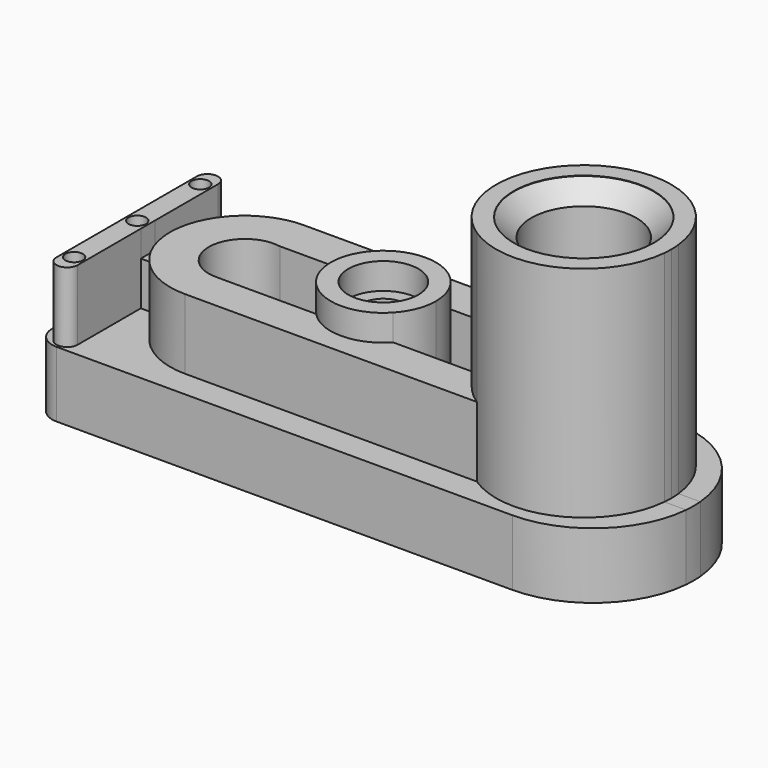
from build123d import *

# Parameters (mm, degrees)
F1_DEPTH  = 15
F0_R      = 2
F2_DEPTH  = 31
F3_DEPTH  = 25
F4_DEPTH  = 31
F0_R_2    = 8
F5_DEPTH  = 37
F0_R_3    = 5
F6_DEPTH  = 31
F0_R_4    = 16
F0_R_5    = 12
F7_DEPTH  = 65
F8_DEPTH  = 65
F10_DEPTH = 15
F11_DEPTH = 15


# Not quite as in the source:
# - a fillet or chamfer that OpenCascade refuses, or shapes differently, is made with other operations: its cross-section is extruded or revolved along the edge and cut away or added
# - a feature names something its author has since deleted; it is built from what else it names


with BuildPart() as f1:
    # F0 (on Top) → F1 (new body)
    with BuildSketch(Plane.XY):
        with BuildLine():
            ThreePointArc((77.4165694517, 2), (70.0412743977, 16.9583212199), (54.4963863199, 23.0000763868))
            Line((54.4963863199, 23.0000763868), (-49.5028280384, 23.0000763868))
            ThreePointArc((-49.5028280384, 23.0000763868), (-53.0386396779, 21.5353325374), (-54.5028279767, 17.9992908068))
            Line((-54.5028279767, 17.9992908068), (-54.4971717765, -18.0008619668))
            ThreePointArc((-54.4971717765, -18.0008619668), (-53.0324279887, -21.5358880263), (-49.4971718382, -23.0000763868))
            Line((-49.4971718382, -23.0000763868), (54.5036136801, -23.0000763868))
            ThreePointArc((54.5036136801, -23.0000763868), (70.024037462, -16.9740969207), (77.4118141054, -2.0537504379))
            Line((77.4118141054, -2.0537504379), (72.4417991653, -2.0537504379))
            ThreePointArc((72.4417991653, -2.0537504379), (61.1210212719, -18.2127692775), (41.4420685321, -16.7940652806))
            Line((41.4420685321, -16.7940652806), (-25.1657858694, -16.7940652806))
            ThreePointArc((-25.1657858694, -16.7940652806), (-36.3795967687, -12.5710150384), (-42.0220562758, -2))
            Line((-42.0220562758, -2), (-47.0725483227, -2))
            Line((-47.0725483227, -2), (-47.0801730056, -20.0009441468))
            ThreePointArc((-47.0801730056, -20.0009441468), (-49.4958146373, -22.4147707226), (-51.9095643269, -19.999052265))
            Line((-51.9095643269, -19.999052265), (-51.8926214772, 20.0009441468))
            ThreePointArc((-51.8926214772, 20.0009441468), (-49.4769799058, 22.4146170129), (-47.0632301559, 19.999052265))
            Line((-47.0632301559, 19.999052265), (-47.0708540375, 2))
            Line((-47.0708540375, 2), (-42.0708540375, 2))
            ThreePointArc((-42.0708540375, 2), (-36.5346224464, 12.8451417707), (-25.1657858694, 17.2059347194))
            Line((-25.1657858694, 17.2059347194), (42.5953938554, 17.2059347194))
            ThreePointArc((42.5953938554, 17.2059347194), (61.6177075826, 17.6666940031), (72.4165694517, 2))
            Line((72.4165694517, 2), (77.4165694517, 2))
        make_face()
    extrude(amount=F1_DEPTH)

    # F0 (on Top) → F2 (join)
    with BuildSketch(Plane.XY):
        with BuildLine():
            Line((-47.0725483227, -2), (-47.0708540375, 2))
            Line((-47.0708540375, 2), (-47.0632301559, 19.999052265))
            ThreePointArc((-47.0632301559, 19.999052265), (-49.4769799058, 22.4146170129), (-51.8926214772, 20.0009441468))
            Line((-51.8926214772, 20.0009441468), (-51.9095643269, -19.999052265))
            ThreePointArc((-51.9095643269, -19.999052265), (-49.4958146373, -22.4147707226), (-47.0801730056, -20.0009441468))
            Line((-47.0801730056, -20.0009441468), (-47.0725483227, -2))
        make_face()
        with Locations((-49.4971718382, -18.0000763868)):
            Circle(F0_R, mode=Mode.SUBTRACT)
        with Locations((-49.4863972414, 0)):
            Circle(F0_R, mode=Mode.SUBTRACT)
        with Locations((-49.5028280384, 18.0000763868)):
            Circle(F0_R, mode=Mode.SUBTRACT)
    extrude(amount=F2_DEPTH)

    # F0 (on Top) → F3 (join)
    with BuildSketch(Plane.XY):
        with BuildLine():
            ThreePointArc((-42.0220562758, -2), (-42.1645209866, -0.0014403371), (-42.0708540375, 2))
            Line((-42.0708540375, 2), (-47.0708540375, 2))
            Line((-47.0708540375, 2), (-47.0725483227, -2))
            Line((-47.0725483227, -2), (-42.0220562758, -2))
        make_face()
    extrude(amount=F3_DEPTH)

    # F0 (on Top) → F4 (join)
    with BuildSketch(Plane.XY):
        with BuildLine():
            ThreePointArc((34.3503431001, 8.1804120839), (37.766383698, 13.3385657076), (42.5953938554, 17.2059347194))
            Line((42.5953938554, 17.2059347194), (-25.1657858694, 17.2059347194))
            ThreePointArc((-25.1657858694, 17.2059347194), (-36.5346224464, 12.8451417707), (-42.0708540375, 2))
            ThreePointArc((-42.0708540375, 2), (-42.1645209866, -0.0014403371), (-42.0220562758, -2))
            ThreePointArc((-42.0220562758, -2), (-36.3795967687, -12.5710150384), (-25.1657858694, -16.7940652806))
            Line((-25.1657858694, -16.7940652806), (41.4420685321, -16.7940652806))
            ThreePointArc((41.4420685321, -16.7940652806), (37.2108856838, -13.0055426049), (34.2152341998, -8.1804120839))
            Line((34.2152341998, -8.1804120839), (15.4548283117, -8.1804120839))
            ThreePointArc((15.4548283117, -8.1804120839), (6.6752578132, -12), (-2.1043126853, -8.1804120839))
            Line((-2.1043126853, -8.1804120839), (-24.9639281544, -8.1804120839))
            ThreePointArc((-24.9639281544, -8.1804120839), (-33.1770221677, 0.8003828075), (-23.5, 8.1804120839))
            Line((-23.5, 8.1804120839), (-2.1043126853, 8.1804120839))
            ThreePointArc((-2.1043126853, 8.1804120839), (6.6752578132, 12), (15.4548283117, 8.1804120839))
            Line((15.4548283117, 8.1804120839), (34.3503431001, 8.1804120839))
        make_face()
    extrude(amount=F4_DEPTH)

    # F0 (on Top) → F5 (join)
    with BuildSketch(Plane.XY):
        with BuildLine():
            ThreePointArc((18.6752578132, 0), (17.8411622992, 4.3957453303), (15.4548283117, 8.1804120839))
            ThreePointArc((15.4548283117, 8.1804120839), (6.6752578132, 12), (-2.1043126853, 8.1804120839))
            ThreePointArc((-2.1043126853, 8.1804120839), (-5.3247421868, 0), (-2.1043126853, -8.1804120839))
            ThreePointArc((-2.1043126853, -8.1804120839), (6.6752578132, -12), (15.4548283117, -8.1804120839))
            ThreePointArc((15.4548283117, -8.1804120839), (17.8411622992, -4.3957453303), (18.6752578132, 0))
        make_face()
        with Locations((6.6752578132, 0)):
            Circle(F0_R_2, mode=Mode.SUBTRACT)
    extrude(amount=F5_DEPTH)

    # F0 (on Top) → F6 (join)
    with BuildSketch(Plane.XY):
        with Locations((6.6752578132, 0)):
            Circle(F0_R_2)
        with Locations((6.6752578132, 0)):
            Circle(F0_R_3, mode=Mode.SUBTRACT)
    extrude(amount=F6_DEPTH)


with BuildPart() as f7:
    # F0 (on Top) → F7 (new body)
    with BuildSketch(Plane.XY):
        with Locations((52.5325443108, -0.1507078368)):
            Circle(F0_R_4)
        with Locations((52.5325443108, -0.1507078368)):
            Circle(F0_R_5, mode=Mode.SUBTRACT)
    extrude(amount=F7_DEPTH)

    # F9: chamfer of 4.1 on 1 edges, made by hand

    # F9_s1 → F9_t2 (revolve, cut)
    with BuildSketch(Plane.XZ.offset(0.1507078368)):
        Polygon((64.5325443108, 60.9), (68.6325443108, 65), (64.5325443108, 65), align=None)
    revolve(axis=Axis((52.5325443108, -0.1507078368, 65), (0, 0, 1)), mode=Mode.SUBTRACT)


with BuildPart() as f8:
    # F0 (on Top) → F8 (new body)
    with BuildSketch(Plane.XY):
        with BuildLine():
            ThreePointArc((72.5325443108, -0.1507078368), (72.5035295496, 0.926208405), (72.4165694517, 2))
            ThreePointArc((72.4165694517, 2), (61.6177075826, 17.6666940031), (42.5953938554, 17.2059347194))
            ThreePointArc((42.5953938554, 17.2059347194), (37.766383698, 13.3385657076), (34.3503431001, 8.1804120839))
            ThreePointArc((34.3503431001, 8.1804120839), (32.5332262339, 0.0144480163), (34.2152341998, -8.1804120839))
            ThreePointArc((34.2152341998, -8.1804120839), (37.2108856838, -13.0055426049), (41.4420685321, -16.7940652806))
            ThreePointArc((41.4420685321, -16.7940652806), (61.1210212719, -18.2127692775), (72.4417991653, -2.0537504379))
            ThreePointArc((72.4417991653, -2.0537504379), (72.5098451431, -1.1033103015), (72.5325443108, -0.1507078368))
        make_face()
        with Locations((52.5325443108, -0.1507078368)):
            Circle(F0_R_4, mode=Mode.SUBTRACT)
    extrude(amount=F8_DEPTH)


with BuildPart() as f10:
    # F0 (on Top) → F10 (new body)
    with BuildSketch(Plane.XY):
        with BuildLine():
            ThreePointArc((-2.1043126853, -8.1804120839), (-5.3247421868, 0), (-2.1043126853, 8.1804120839))
            Line((-2.1043126853, 8.1804120839), (-23.5, 8.1804120839))
            ThreePointArc((-23.5, 8.1804120839), (-33.1770221677, 0.8003828075), (-24.9639281544, -8.1804120839))
            Line((-24.9639281544, -8.1804120839), (-2.1043126853, -8.1804120839))
        make_face()
    extrude(amount=F10_DEPTH)


with BuildPart() as f10b:
    # F0 (on Top) → F10, piece 2 (new body)
    with BuildSketch(Plane.XY):
        with BuildLine():
            ThreePointArc((34.2152341998, -8.1804120839), (32.5332262339, 0.0144480163), (34.3503431001, 8.1804120839))
            Line((34.3503431001, 8.1804120839), (15.4548283117, 8.1804120839))
            ThreePointArc((15.4548283117, 8.1804120839), (17.8411622992, 4.3957453303), (18.6752578132, 0))
            ThreePointArc((18.6752578132, 0), (17.8411622992, -4.3957453303), (15.4548283117, -8.1804120839))
            Line((15.4548283117, -8.1804120839), (34.2152341998, -8.1804120839))
        make_face()
    extrude(amount=F10_DEPTH)


with BuildPart() as f11:
    # F0 (on Top) → F11 (new body)
    with BuildSketch(Plane.XY):
        with BuildLine():
            ThreePointArc((77.4118141054, -2.0537504379), (77.5036748095, -0.0269801891), (77.4165694517, 2))
            Line((77.4165694517, 2), (72.4165694517, 2))
            ThreePointArc((72.4165694517, 2), (72.5035295496, 0.926208405), (72.5325443108, -0.1507078368))
            ThreePointArc((72.5325443108, -0.1507078368), (72.5098451431, -1.1033103015), (72.4417991653, -2.0537504379))
            Line((72.4417991653, -2.0537504379), (77.4118141054, -2.0537504379))
        make_face()
    extrude(amount=F11_DEPTH)


solid = Compound([f1.part, f7.part, f8.part, f10.part, f10b.part, f11.part])
